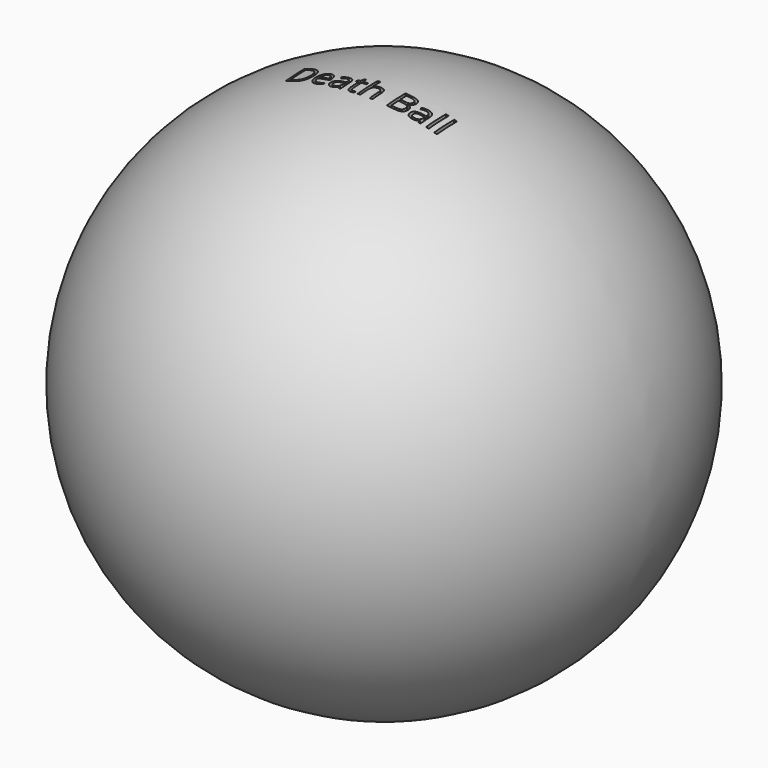
from build123d import *

# Parameters (mm, degrees)
F2_TEXT_SIZE = 9.4878545497
F3_DEPTH     = 177.8


# Not quite as in the source:
# - Text() gives the source's letters only with a copy of the font that has no kerning and outlines rounded to 1/6400 em; it was checked with that copy


with BuildPart() as f1:
    # F0 (on Front) → F1 (revolve)
    with BuildSketch(Plane.XZ):
        with BuildLine():
            Line((0, 76.2), (0, -76.2))
            ThreePointArc((0, -76.2), (76.2, 0), (0, 76.2))
        make_face()
    revolve(axis=Axis((0, 0, 0), (0, 0, -1)))

    # F2 (on Top) → F3 (cut)
    with BuildSketch(Plane.XY):
        with Locations((-23.8118134439, -6.8312552758)):
            Text('Death Ball', F2_TEXT_SIZE, font='Open Sans', text_align=(TextAlign.LEFT, TextAlign.BOTTOM))
    extrude(amount=F3_DEPTH, mode=Mode.SUBTRACT)


solid = f1.part
